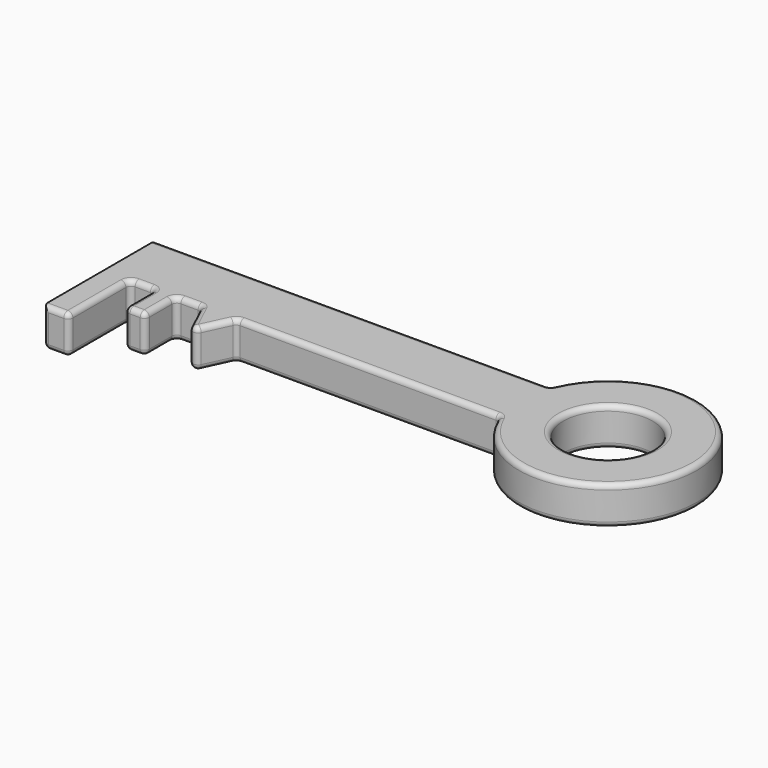
from build123d import *

# Parameters (mm, degrees)
F0_R     = 17.5
F0_W     = 10
F0_H     = 30
F0_W_2   = 8
F0_H_2   = 15
F1_DEPTH = 15
F2_R     = 2


with BuildPart() as f1:
    # F0 (on Top) → F1 (new body)
    with BuildSketch(Plane.XY):
        Polygon((67.5656899738, 22.5906066601), (-87.4343100262, 22.5906066601), (-87.4343100262, -2.4093933399), (-77.4343100262, -2.4093933399), (-67.4343100262, -2.4093933399), (-59.4343100262, -2.4093933399), (-49.4343100262, -2.4093933399), (-35.4343100262, -2.4093933399), (67.5656899738, -2.4093933399), align=None)
        with BuildLine():
            ThreePointArc((67.5656899738, -2.4093933399), (135.2574320504, 10.0906066601), (67.5656899738, 22.5906066601))
            Line((67.5656899738, 22.5906066601), (67.5656899738, -2.4093933399))
        make_face()
        with Locations((100.2574320504, 10.0906066601)):
            Circle(F0_R, mode=Mode.SUBTRACT)
        with Locations((-82.4343100262, -17.4093933399)):
            Rectangle(F0_W, F0_H)
        Polygon((-42.4343100262, -17.4094536398), (-35.4343100262, -2.4093933399), (-49.4343100262, -2.4093933399), align=None)
        with Locations((-63.4343100262, -9.9093933399)):
            Rectangle(F0_W_2, F0_H_2)
    extrude(amount=F1_DEPTH)

    # F2
    f2_edges = [f1.edges().sort_by_distance(p)[0] for p in [
        (-35.43431, -2.409393, 7.5),
        (-45.93431, -9.909423, 0),
        (-59.43431, -17.409393, 7.5),
        (-49.43431, -2.409393, 7.5),
        (-67.43431, -17.409393, 7.5),
        (-42.43431, -17.409454, 7.5),
        (-45.93431, -9.909423, 15),
        (-38.93431, -9.909423, 0),
        (-87.43431, -4.909393, 0),
        (135.257432, 10.090607, 0),
        (135.257432, 10.090607, 15),
        (82.757432, 10.090607, 0),
        (82.757432, 10.090607, 15),
        (-77.43431, -17.409393, 0),
        (-87.43431, 22.590607, 7.5),
        (-72.43431, -2.409393, 0),
        (-59.43431, -2.409393, 7.5),
        (67.56569, -2.409393, 7.5),
        (-54.43431, -2.409393, 0),
        (-9.93431, 22.590607, 0),
        (-9.93431, 22.590607, 15),
        (67.56569, 22.590607, 7.5),
        (-77.43431, -2.409393, 7.5),
        (-59.43431, -9.909393, 15),
        (-72.43431, -2.409393, 15),
        (-54.43431, -2.409393, 15),
        (-67.43431, -9.909393, 0),
        (-67.43431, -9.909393, 15),
        (-59.43431, -9.909393, 0),
        (16.06569, -2.409393, 0),
        (16.06569, -2.409393, 15),
        (-38.93431, -9.909423, 15),
        (-82.43431, -32.409393, 0),
        (-63.43431, -17.409393, 0),
        (-63.43431, -17.409393, 15),
        (-67.43431, -2.409393, 7.5),
        (-87.43431, -32.409393, 7.5),
        (-82.43431, -32.409393, 15),
        (-77.43431, -32.409393, 7.5),
        (-77.43431, -17.409393, 15),
    ]]
    fillet(f2_edges, radius=F2_R)


solid = f1.part
